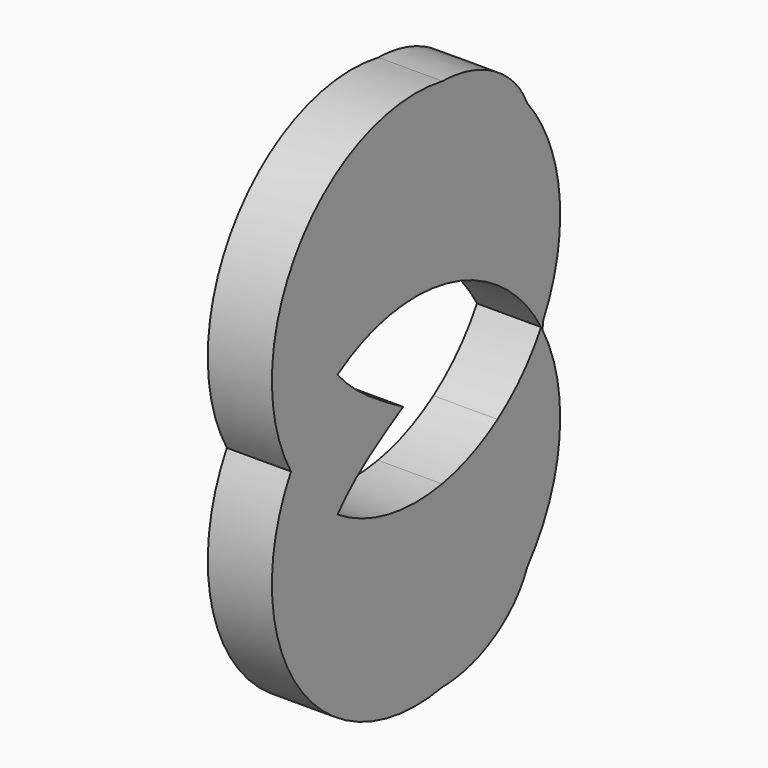
from build123d import *

# Parameters (mm, degrees)
F1_DEPTH = 25.4


with BuildPart() as f1:
    # F0 (on Right) → F1 (new body)
    with BuildSketch(Plane.YZ):
        with BuildLine():
            ThreePointArc((77.7355076163, 35.4636907578), (76.6675961502, 47.7624663657), (73.4958271318, 59.6931074906))
            Line((73.4958271318, 59.6931074906), (69.2378436874, 1.6926861527))
            ThreePointArc((69.2378436874, 1.6926861527), (75.5784886533, 18.0518338473), (77.7355076163, 35.4636907578))
        make_face()
        with BuildLine():
            Line((69.2378436874, 1.6926861527), (73.4958271318, 59.6931074906))
            ThreePointArc((73.4958271318, 59.6931074906), (68.3879297776, 70.7709703077), (61.4677361542, 80.8168938687))
            add(Edge.make_bspline(
                [(46.7271482261, 23.3890579279), (57.3671713501, 38.6358972227), (67.4277924366, 61.0196278452), (62.6176115866, 78.1431138882), (61.4677361542, 80.8168938687)],
                knots=[0.2275291842, 0.2275291842, 0.2275291842, 0.2275291842, 0.3610428006, 0.3876214238, 0.3876214238, 0.3876214238, 0.3876214238], degree=3))
            ThreePointArc((46.7271482261, 23.3890579279), (58.8331802448, 12.9122292433), (68.2986060932, 0))
            ThreePointArc((68.2986060932, 0), (68.7739653696, 0.8431577995), (69.2378436874, 1.6926861527))
        make_face()
        with BuildLine():
            Line((69.0189883561, -1.2884671556), (69.2378436874, 1.6926861527))
            ThreePointArc((69.2378436874, 1.6926861527), (68.7739653696, 0.8431577995), (68.2986060932, 0))
            ThreePointArc((68.2986060932, 0), (68.6621292842, -0.6423706226), (69.0189883561, -1.2884671556))
        make_face()
        with BuildLine():
            add(Edge.make_bspline(
                [(46.7271482261, 23.3890579279), (57.3671713501, 38.6358972227), (67.4277924366, 61.0196278452), (62.6176115866, 78.1431138882), (61.4677361542, 80.8168938687)],
                knots=[0.2275291842, 0.2275291842, 0.2275291842, 0.2275291842, 0.3610428006, 0.3876214238, 0.3876214238, 0.3876214238, 0.3876214238], degree=3))
            ThreePointArc((61.4677361542, 80.8168938687), (42.6716941747, 96.9001796523), (19.5137307938, 105.5991455529))
            add(Edge.make_bspline(
                [(19.5137307938, 105.5991455529), (15.2484459589, 105.6418292249), (-17.4670589129, 101.9834872227), (-51.4356414133, 56.0713753865), (-36.7498246069, 29.4728703431), (-32.4913798704, 24.3725458831)],
                knots=[0.5361274609, 0.5361274609, 0.5361274609, 0.5361274609, 0.5710508717, 0.8014313121, 0.8647451677, 0.8647451677, 0.8647451677, 0.8647451677], degree=3))
            ThreePointArc((-32.4913798704, 24.3725458831), (-6.4015352071, 34.736385461), (21.6668981331, 34.2341751698))
            ThreePointArc((21.6668981331, 34.2341751698), (34.7206440257, 30.0215683701), (46.7271482261, 23.3890579279))
        make_face()
        with BuildLine():
            ThreePointArc((19.5137307938, 105.5991455529), (42.6716941747, 96.9001796523), (61.4677361542, 80.8168938687))
            add(Edge.make_bspline(
                [(61.4677361542, 80.8168938687), (55.0428945656, 95.7564363048), (37.6511501332, 105.4176402871), (19.5137307938, 105.5991455529)],
                knots=[0.3876214238, 0.3876214238, 0.3876214238, 0.3876214238, 0.5361274609, 0.5361274609, 0.5361274609, 0.5361274609], degree=3))
        make_face()
        with BuildLine():
            ThreePointArc((77.7355076163, -35.4636907578), (75.5220462625, -17.829040093), (69.0189883561, -1.2884671556))
            Line((69.0189883561, -1.2884671556), (64.0810679537, -68.550697648))
            add(Edge.make_bspline(
                [(64.0810679537, -68.550697648), (64.055573163, -69.8265995508), (63.9650070893, -71.0818079643), (63.8049086741, -72.3124207221)],
                knots=[0.3500957655, 0.3500957655, 0.3500957655, 0.3500957655, 0.3610428006, 0.3610428006, 0.3610428006, 0.3610428006], degree=3))
            add(Edge.make_bspline(
                [(63.8049086741, -72.3124207221), (63.4162011029, -75.3002610177), (62.6176115866, -78.1431138882), (61.4677361542, -80.8168938687)],
                knots=[0.3610428006, 0.3610428006, 0.3610428006, 0.3610428006, 0.3876214238, 0.3876214238, 0.3876214238, 0.3876214238], degree=3))
            ThreePointArc((61.4677361542, -80.8168938687), (73.5455465545, -59.5549413519), (77.7355076163, -35.4636907578))
        make_face()
        with BuildLine():
            Line((64.0810679537, -68.550697648), (69.0189883561, -1.2884671556))
            ThreePointArc((69.0189883561, -1.2884671556), (68.6621292842, -0.6423706226), (68.2986060932, 0))
            ThreePointArc((68.2986060932, 0), (58.8331802447, -12.9122292433), (46.7271482261, -23.3890579279))
            add(Edge.make_bspline(
                [(46.7271482261, -23.3890579279), (56.4947756325, -37.3857798919), (64.3665159576, -54.2652831945), (64.0810679537, -68.550697648)],
                knots=[0.2275291842, 0.2275291842, 0.2275291842, 0.2275291842, 0.3500957655, 0.3500957655, 0.3500957655, 0.3500957655], degree=3))
        make_face()
        with BuildLine():
            add(Edge.make_bspline(
                [(19.5137307938, 105.5991455529), (15.2484459589, 105.6418292249), (-17.4670589129, 101.9834872227), (-51.4356414133, 56.0713753865), (-36.7498246069, 29.4728703431), (-32.4913798704, 24.3725458831)],
                knots=[0.5361274609, 0.5361274609, 0.5361274609, 0.5361274609, 0.5710508717, 0.8014313121, 0.8647451677, 0.8647451677, 0.8647451677, 0.8647451677], degree=3))
            ThreePointArc((19.5137307938, 105.5991455529), (-51.7805921013, 76.7996475885), (-55.5363464012, 0))
            ThreePointArc((-55.5363464012, 0), (-45.4663442086, 13.5596369664), (-32.4913798704, 24.3725458831))
        make_face()
        with BuildLine():
            Line((63.8049086741, -72.3124207222), (64.0810679537, -68.550697648))
            add(Edge.make_bspline(
                [(46.7271482261, -23.3890579279), (56.4947756325, -37.3857798919), (64.3665159576, -54.2652831945), (64.0810679537, -68.550697648)],
                knots=[0.2275291842, 0.2275291842, 0.2275291842, 0.2275291842, 0.3500957655, 0.3500957655, 0.3500957655, 0.3500957655], degree=3))
            ThreePointArc((46.7271482261, -23.3890579279), (33.6000701349, -30.4952094493), (19.2818065466, -34.7147943189))
            ThreePointArc((19.2818065466, -34.7147943189), (-7.5965149208, -34.5082512887), (-32.4913798704, -24.3725458831))
            add(Edge.make_bspline(
                [(19.5137307938, -105.5991455529), (15.2484459589, -105.6418292249), (-17.4670589129, -101.9834872227), (-51.4356414133, -56.0713753865), (-36.7498246069, -29.4728703431), (-32.4913798704, -24.3725458831)],
                knots=[0.5361274609, 0.5361274609, 0.5361274609, 0.5361274609, 0.5710508717, 0.8014313121, 0.8647451677, 0.8647451677, 0.8647451677, 0.8647451677], degree=3))
            ThreePointArc((19.5137307938, -105.5991455529), (42.6716941747, -96.9001796523), (61.4677361542, -80.8168938687))
            add(Edge.make_bspline(
                [(63.8049086741, -72.3124207221), (63.4162011029, -75.3002610177), (62.6176115866, -78.1431138882), (61.4677361542, -80.8168938687)],
                knots=[0.3610428006, 0.3610428006, 0.3610428006, 0.3610428006, 0.3876214238, 0.3876214238, 0.3876214238, 0.3876214238], degree=3))
        make_face()
        with BuildLine():
            ThreePointArc((-32.4913798704, 24.3725458831), (-45.4663442086, 13.5596369664), (-55.5363464012, 0))
            ThreePointArc((-55.5363464012, 0), (-45.4663442086, -13.5596369664), (-32.4913798704, -24.3725458831))
            add(Edge.make_bspline(
                [(-32.4913798704, -24.3725458831), (-23.3942363951, -13.4769287613), (-9.3112886841, -5.4733246177), (0, 0)],
                knots=[0.8647451677, 0.8647451677, 0.8647451677, 0.8647451677, 1, 1, 1, 1], degree=3))
            add(Edge.make_bspline(
                [(-32.4913798704, 24.3725458831), (-23.3942363951, 13.4769287613), (-9.3112886841, 5.4733246177), (0, 0)],
                knots=[0.8647451677, 0.8647451677, 0.8647451677, 0.8647451677, 1, 1, 1, 1], degree=3))
        make_face()
        with BuildLine():
            ThreePointArc((-32.4913798704, -24.3725458831), (-45.4663442086, -13.5596369664), (-55.5363464012, 0))
            ThreePointArc((-55.5363464012, 0), (-51.7805921013, -76.7996475885), (19.5137307938, -105.5991455529))
            add(Edge.make_bspline(
                [(19.5137307938, -105.5991455529), (15.2484459589, -105.6418292249), (-17.4670589129, -101.9834872227), (-51.4356414133, -56.0713753865), (-36.7498246069, -29.4728703431), (-32.4913798704, -24.3725458831)],
                knots=[0.5361274609, 0.5361274609, 0.5361274609, 0.5361274609, 0.5710508717, 0.8014313121, 0.8647451677, 0.8647451677, 0.8647451677, 0.8647451677], degree=3))
        make_face()
        with BuildLine():
            add(Edge.make_bspline(
                [(61.4677361542, -80.8168938687), (55.0428945656, -95.7564363048), (37.6511501332, -105.4176402871), (19.5137307938, -105.5991455529)],
                knots=[0.3876214238, 0.3876214238, 0.3876214238, 0.3876214238, 0.5361274609, 0.5361274609, 0.5361274609, 0.5361274609], degree=3))
            ThreePointArc((61.4677361542, -80.8168938687), (42.6716941747, -96.9001796523), (19.5137307938, -105.5991455529))
        make_face()
    extrude(amount=F1_DEPTH)


solid = f1.part
